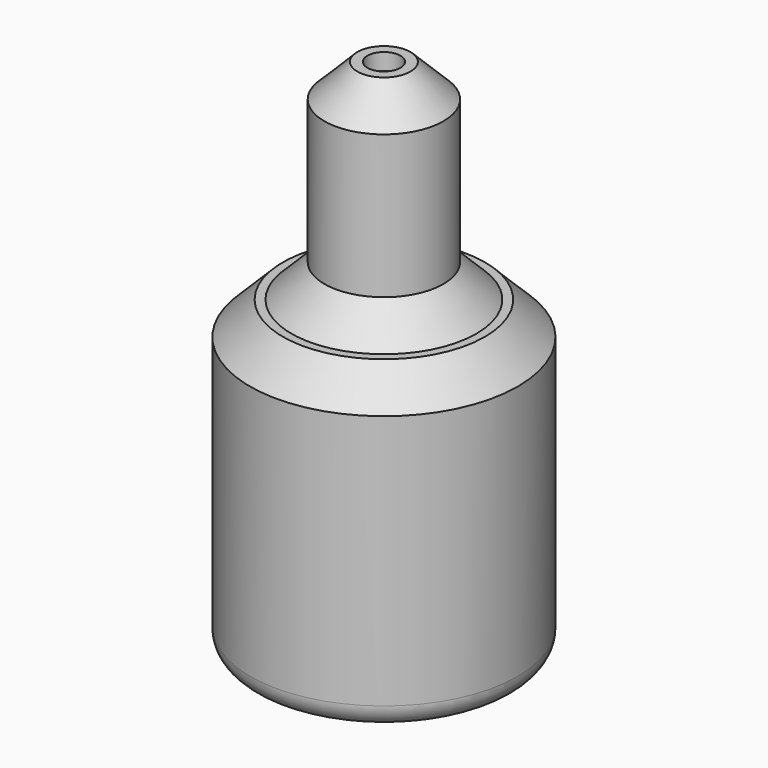
from build123d import *

# Parameters (mm, degrees)
F0_R           = 18.0428144426
F1_DEPTH       = 63.5
F2_W           = 40.2940958738
F2_H           = 94.3237841129
F4_SIZE        = 10
F6_D           = 5
F6_CBORE_D     = 10
F6_CBORE_DEPTH = 5
F7_R           = 7
F8_T           = -2.5


# Not quite as in the source:
# - a shell that OpenCascade refuses in one call is made with other operations: the cavity is built on its own and cut out


with BuildPart() as f1:
    # F0 (on Top) → F1 (new body, symmetric)
    with BuildSketch(Plane.XY):
        Circle(F0_R)
    extrude(amount=F1_DEPTH, both=True)

    # F2 (on Front) → F3 (revolve)
    with BuildSketch(Plane.XZ):
        with Locations((20.4668417573, -47.1034049988)):
            Rectangle(F2_W, F2_H)
    revolve(axis=Axis((0, 0, 0), (0, 0, 1)))

    # F4
    f4_edges = [f1.edges().sort_by_distance(p)[0] for p in [
        (-40.61389, 0, 0.058487),
        (-18.042814, 0, 0.058487),
        (18.042814, 0, 31.779244),
        (-18.042814, 0, 63.5),
    ]]
    chamfer(f4_edges, length=F4_SIZE)

    # F6 (through all)
    with Locations(Plane.XY.offset(63.5)):
        with Locations((0, 0)):
            CounterBoreHole(F6_D / 2, F6_CBORE_D / 2, F6_CBORE_DEPTH)

    # F7
    f7_edges = [f1.edges().sort_by_distance(p)[0] for p in [
        (-40.61389, 0, -94.265297),
    ]]
    fillet(f7_edges, radius=F7_R)

    # F8: a shell. OpenCascade refuses it in one call, so the cavity is built on its own and cut out:
    # the body offset inwards by the wall thickness, plus a prism from it out through each open face.
    f8_core = offset(f1.part, amount=F8_T, kind=Kind.INTERSECTION, mode=Mode.PRIVATE)
    f8_exits = [f8_core.faces().sort_by_distance(p)[0] for p in [
        (-5.950744, 0, -91.765297),
    ]]
    add(f8_core, mode=Mode.SUBTRACT)
    extrude(f8_exits, amount=-F8_T, mode=Mode.SUBTRACT)


solid = f1.part
